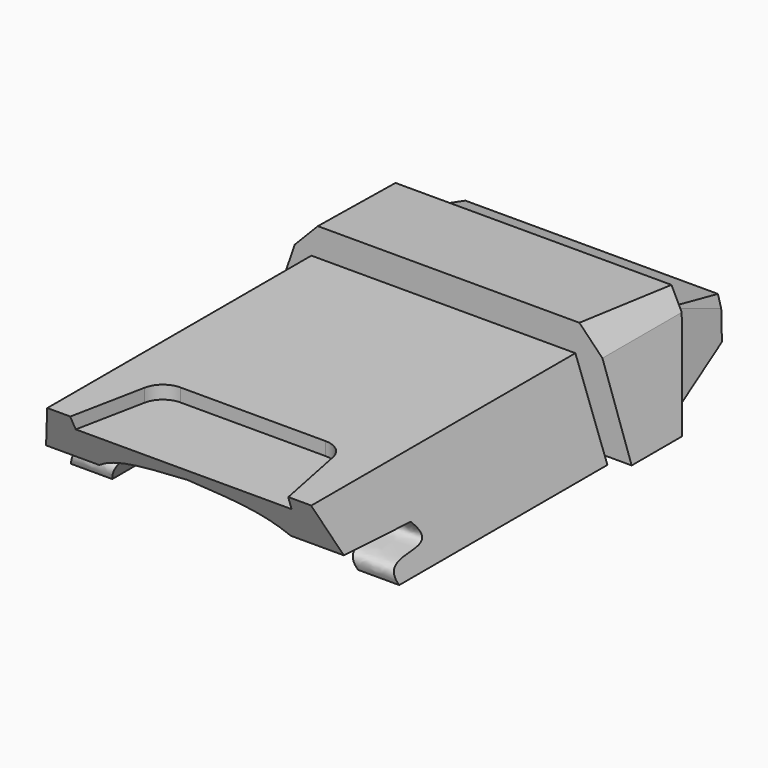
from build123d import *

# Parameters (mm, degrees)
F1_DEPTH               = 25.4
DRAFT_F1_DRAFTED_ANGLE = -20
F2_W                   = 28.2977861404
F2_H                   = 22.5983016491
F3_DEPTH               = 36.068
F5_DEPTH               = 57.658
F7_DEPTH               = 118.872
F8_DEPTH               = 3.81
F10_DEPTH              = 63.754
F12_DEPTH              = 54.102
F14_DEPTH              = 37.846
F16_DEPTH              = 51.054
F18_DEPTH              = 46.736
F20_DEPTH              = 25.4
F22_DEPTH              = 25.4


# Not quite as in the source:
# - an extrude with a draft is written as a straight extrude whose walls are then drafted


with BuildPart() as f1:
    # F0 (on Top) → F1 (new body)
    with BuildSketch(Plane.XY):
        with BuildLine():
            Line((38.1, -47.625), (38.1, 47.625))
            Line((38.1, 47.625), (-38.1, 47.625))
            Line((-38.1, 47.625), (-38.1, -47.625))
            Line((-38.1, -47.625), (-31.4568579197, -47.625))
            Line((-31.4568579197, -47.625), (-27.165672787, -26.1562607157))
            ThreePointArc((-27.165672787, -26.1562607157), (-24.9649539697, -22.4903919131), (-20.9388425957, -21.0508834571))
            Line((-20.9388425957, -21.0508834571), (0, -21.0508834571))
            Line((0, -21.0508834571), (20.9388425957, -21.0508834571))
            ThreePointArc((20.9388425957, -21.0508834571), (24.9649539697, -22.4903919131), (27.165672787, -26.1562607157))
            Line((27.165672787, -26.1562607157), (31.4568579197, -47.625))
            Line((31.4568579197, -47.625), (38.1, -47.625))
        make_face()
        with BuildLine():
            Line((-31.4568579197, -47.625), (31.4568579197, -47.625))
            Line((31.4568579197, -47.625), (27.165672787, -26.1562607157))
            ThreePointArc((27.165672787, -26.1562607157), (24.9649539697, -22.4903919131), (20.9388425957, -21.0508834571))
            Line((20.9388425957, -21.0508834571), (0, -21.0508834571))
            Line((0, -21.0508834571), (-20.9388425957, -21.0508834571))
            ThreePointArc((-20.9388425957, -21.0508834571), (-24.9649539697, -22.4903919131), (-27.165672787, -26.1562607157))
            Line((-27.165672787, -26.1562607157), (-31.4568579197, -47.625))
        make_face()
    extrude(amount=-F1_DEPTH)

    # draft_F1_drafted
    draft_f1_drafted_walls = [f1.faces().sort_by_distance(p)[0] for p in [
        (38.1, 0, -16.9333333333),
        (0, 47.625, -16.9333333333),
        (-38.1, 0, -16.9333333333),
        (0, -47.625, -16.9333333333),
    ]]
    draft(draft_f1_drafted_walls, neutral_plane=Plane(origin=(0, 0, 0), x_dir=(1, 0, 0), z_dir=(0, 0, -1)), angle=DRAFT_F1_DRAFTED_ANGLE)

    # F2 (on face) → F3 (cut)
    with BuildSketch(Plane.XY):
        Polygon((38.1, -47.625), (-38.1, -47.625), (-38.1, -70.2233016491), (69.2304000258, -70.2233016491), (69.2304000258, -47.625), align=None)
        with Locations((-52.2488930702, -58.9241508245)):
            Rectangle(F2_W, F2_H)
        Polygon((-53.3912964165, 69.2494660616), (-53.3912964165, 47.625), (-38.1, 47.625), (38.1, 47.625), (63.4635314345, 47.625), (63.4635314345, 69.2494660616), align=None)
    extrude(amount=-F3_DEPTH, mode=Mode.SUBTRACT)

    # F4 (on Right) → F5 (cut, symmetric)
    with BuildSketch(Plane.YZ):
        with BuildLine():
            Line((-18.3125212789, -14.3378842622), (-48.1080040336, -13.109754771))
            Line((-48.1080040336, -13.109754771), (-48.6956569099, -27.3667213753))
            Line((-48.6956569099, -27.3667213753), (-27.3366011679, -25.6580319256))
            add(Edge.make_bspline(
                [(-18.3125212789, -14.3378842622), (-8.8612670079, -24.8036812991), (-32.676294446, -15.5660128221), (-27.3366011679, -25.6580319256)],
                knots=[0, 0, 0, 0, 14.4768698607, 14.4768698607, 14.4768698607, 14.4768698607], degree=3))
        make_face()
    extrude(amount=F5_DEPTH, both=True, mode=Mode.SUBTRACT)

    # F6 (on face) → F7 (cut)
    with BuildSketch(Plane(origin=(0, 47.625, 0), x_dir=(-1, 0, 0), z_dir=(0, 1, 0))):
        with BuildLine():
            Line((-33.061414957, -18.7426097691), (-35.484506839, -25.4))
            Line((-35.484506839, -25.4), (35.484506839, -25.4))
            Line((35.484506839, -25.4), (33.061414957, -18.7426097691))
            add(Edge.make_bspline(
                [(33.061414957, -18.7426097691), (25.6499633823, -9.0257734998), (16.5739841759, -8.4904003888), (0, -7.1020801552)],
                knots=[0, 0, 0, 0, 35.0508072468, 35.0508072468, 35.0508072468, 35.0508072468], degree=3))
            add(Edge.make_bspline(
                [(-33.061414957, -18.7426097691), (-25.6499633823, -9.0257734998), (-16.5739841759, -8.4904003888), (0, -7.1020801552)],
                knots=[0, 0, 0, 0, 35.0508072468, 35.0508072468, 35.0508072468, 35.0508072468], degree=3))
        make_face()
    extrude(amount=-F7_DEPTH, mode=Mode.SUBTRACT)

    # F0 (on Top) → F8 (cut)
    with BuildSketch(Plane.XY):
        with BuildLine():
            Line((-31.4568579197, -47.625), (31.4568579197, -47.625))
            Line((31.4568579197, -47.625), (27.165672787, -26.1562607157))
            ThreePointArc((27.165672787, -26.1562607157), (24.9649539697, -22.4903919131), (20.9388425957, -21.0508834571))
            Line((20.9388425957, -21.0508834571), (0, -21.0508834571))
            Line((0, -21.0508834571), (-20.9388425957, -21.0508834571))
            ThreePointArc((-20.9388425957, -21.0508834571), (-24.9649539697, -22.4903919131), (-27.165672787, -26.1562607157))
            Line((-27.165672787, -26.1562607157), (-31.4568579197, -47.625))
        make_face()
    extrude(amount=-F8_DEPTH, mode=Mode.SUBTRACT)

    # F9 (on Right) → F10 (cut, symmetric)
    with BuildSketch(Plane.YZ):
        Polygon((-48.974275589, -14.7424889728), (-41.3385145366, -14.902680181), (-48.974275589, 3.0386860017), align=None)
    extrude(amount=F10_DEPTH, both=True, mode=Mode.SUBTRACT)


with BuildPart() as f12:
    # F11 (on Right) → F12 (new body, symmetric)
    with BuildSketch(Plane.YZ):
        Polygon((49.519021064, 6.8399081888), (49.519021064, 0), (49.519021064, -24.5136488229), (67.6910057664, -24.5136488229), (80.1370069385, 4.696352873), align=None)
    extrude(amount=F12_DEPTH, both=True)

    # F13 (on face) → F14 (cut)
    with BuildSketch(Plane.XZ.offset(-49.519021064)):
        Polygon((-54.102, -24.5136488229), (-52.8350435197, -24.5136488229), (-44.3936027586, 0), (-37.7482138574, 6.8399081888), (-54.102, 6.8399081888), align=None)
        Polygon((44.3936027586, 0), (52.8350435197, -24.5136488229), (54.102, -24.5136488229), (54.102, 6.8399081888), (37.7482138574, 6.8399081888), align=None)
    extrude(amount=-F14_DEPTH, mode=Mode.SUBTRACT)

    # F15 (on face) → F16 (cut)
    with BuildSketch(Plane.XZ.offset(-49.519021064)):
        with BuildLine():
            add(Edge.make_bspline(
                [(-35.3140830994, -24.5136488229), (-29.2729102075, -10.8938058838), (-21.721445024, -9.2324828729), (0, -7.1180728264)],
                knots=[0, 0, 0, 0, 39.3661088933, 39.3661088933, 39.3661088933, 39.3661088933], degree=3))
            Line((-35.3140830994, -24.5136488229), (35.3140830994, -24.5136488229))
            add(Edge.make_bspline(
                [(35.3140830994, -24.5136488229), (29.2729102075, -10.8938058838), (21.721445024, -9.2324828729), (0, -7.1180728264)],
                knots=[0, 0, 0, 0, 39.3661088933, 39.3661088933, 39.3661088933, 39.3661088933], degree=3))
        make_face()
    extrude(amount=-F16_DEPTH, mode=Mode.SUBTRACT)


with BuildPart() as f18:
    # F17 (on Right) → F18 (new body, symmetric)
    with BuildSketch(Plane.YZ):
        Polygon((79.6277672052, -1.568368054), (70.325024426, -24.2659784853), (97.1538648009, -16.4147671312), (101.0806262493, -7.2019794025), align=None)
    extrude(amount=F18_DEPTH, both=True)

    # F19 (on face) → F20 (cut)
    with BuildSketch(Plane(origin=(0, 68.7258863168, -28.167689485), x_dir=(1, 0, 0), z_dir=(0, -0.9252987955, 0.3792388945))):
        Polygon((-46.736, 4.2167038569), (-38.3526310325, 28.7467373365), (-46.736, 28.7467373365), align=None)
        Polygon((46.736, 28.7467373365), (38.3526310325, 28.7467373365), (46.736, 4.2167038569), align=None)
        Polygon((-46.736, 28.7467373365), (-38.3526310325, 28.7467373365), (-35.6349311769, 32.7979065478), (-46.736, 33.8321439922), align=None)
        Polygon((35.9596200287, 32.489027828), (38.3526310325, 28.7467373365), (46.736, 28.7467373365), (51.5385307372, 32.489027828), align=None)
    extrude(amount=-F20_DEPTH, mode=Mode.SUBTRACT)

    # F21 (on face) → F22 (cut)
    with BuildSketch(Plane(origin=(0, 88.1381315141, -37.5670673364), x_dir=(-1, 0, 0), z_dir=(0, 0.9199232839, -0.3920983955))):
        with BuildLine():
            add(Edge.make_bspline(
                [(0, 22.9935480226), (17.9532822222, 22.3166515995), (35.5504948125, 22.9935480226), (35.5428287193, 1.9157211063)],
                knots=[0, 0, 0, 0, 41.3227232994, 41.3227232994, 41.3227232994, 41.3227232994], degree=3))
            add(Edge.make_bspline(
                [(0, 22.9935480226), (-17.9532822222, 22.3166515995), (-35.5504948125, 22.9935480226), (-35.5428287193, 1.9157211063)],
                knots=[0, 0, 0, 0, 41.3227232994, 41.3227232994, 41.3227232994, 41.3227232994], degree=3))
            Line((-35.5428287193, 1.9157211063), (0, 1.9157211063))
            Line((0, 1.9157211063), (35.5428287193, 1.9157211063))
        make_face()
    extrude(amount=-F22_DEPTH, mode=Mode.SUBTRACT)


solid = Compound([f1.part, f12.part, f18.part])
